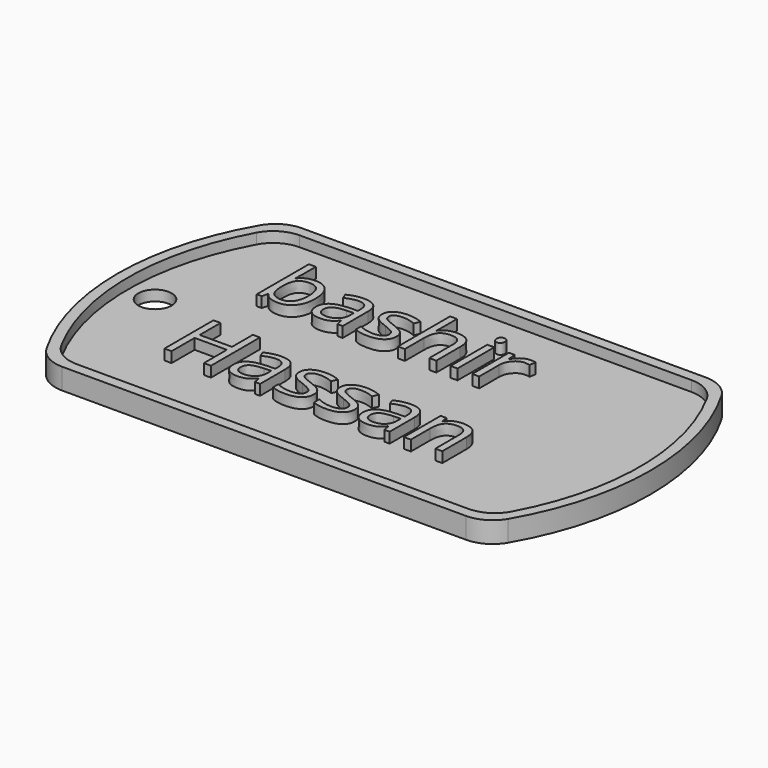
from build123d import *

# Parameters (mm, degrees)
F1_DEPTH     = 1
F3_DEPTH     = 1
F4_R         = 1.5875
F5_DEPTH     = 1
F6_TEXT_SIZE = 8.173513278
F7_DEPTH     = 1


# Not quite as in the source:
# - Text() gives the source's letters only with a copy of the font that has no kerning and outlines rounded to 1/6400 em; it was checked with that copy


with BuildPart() as f1:
    # F0 (on Top) → F1 (new body)
    with BuildSketch(Plane.XY):
        with BuildLine():
            ThreePointArc((-19.2474145991, 14.2875), (-20.8349145991, 13.862130657), (-21.9970452561, 12.7))
            ThreePointArc((-21.9970452561, 12.7), (-25.4, 0), (-21.9970452561, -12.7))
            ThreePointArc((-21.9970452561, -12.7), (-20.8349145991, -13.862130657), (-19.2474145991, -14.2875))
            Line((-19.2474145991, -14.2875), (19.2474145991, -14.2875))
            ThreePointArc((19.2474145991, -14.2875), (20.8349145991, -13.862130657), (21.9970452561, -12.7))
            ThreePointArc((21.9970452561, -12.7), (25.4, 0), (21.9970452561, 12.7))
            ThreePointArc((21.9970452561, 12.7), (20.8349145991, 13.862130657), (19.2474145991, 14.2875))
            Line((19.2474145991, 14.2875), (-19.2474145991, 14.2875))
        make_face()
    extrude(amount=F1_DEPTH)

    # F2 (on face) → F3 (join)
    with BuildSketch(Plane.XY.offset(1)):
        with BuildLine():
            Line((19.2474145991, 14.2875), (-19.2474145991, 14.2875))
            ThreePointArc((-19.2474145991, 14.2875), (-20.8349145991, 13.862130657), (-21.9970452561, 12.7))
            ThreePointArc((-21.9970452561, 12.7), (-25.4, 0), (-21.9970452561, -12.7))
            ThreePointArc((-21.9970452561, -12.7), (-20.8349145991, -13.862130657), (-19.2474145991, -14.2875))
            Line((-19.2474145991, -14.2875), (19.2474145991, -14.2875))
            ThreePointArc((19.2474145991, -14.2875), (20.8349145991, -13.862130657), (21.9970452561, -12.7))
            ThreePointArc((21.9970452561, -12.7), (25.4, 0), (21.9970452561, 12.7))
            ThreePointArc((21.9970452561, 12.7), (20.8349145991, 13.862130657), (19.2474145991, 14.2875))
        make_face()
        with BuildLine():
            ThreePointArc((-21.4526124879, 11.6252061249), (-20.2856017842, 12.8404540819), (-18.6611352482, 13.2875))
            Line((-18.6611352482, 13.2875), (18.6611352482, 13.2875))
            ThreePointArc((18.6611352482, 13.2875), (20.2856017842, 12.8404540819), (21.4526124879, 11.6252061249))
            ThreePointArc((21.4526124879, 11.6252061249), (24.4, 0), (21.4526124879, -11.6252061249))
            ThreePointArc((21.4526124879, -11.6252061249), (20.2856017842, -12.8404540819), (18.6611352482, -13.2875))
            Line((18.6611352482, -13.2875), (-18.6611352482, -13.2875))
            ThreePointArc((-18.6611352482, -13.2875), (-20.2856017842, -12.8404540819), (-21.4526124879, -11.6252061249))
            ThreePointArc((-21.4526124879, -11.6252061249), (-24.4, 0), (-21.4526124879, 11.6252061249))
        make_face(mode=Mode.SUBTRACT)
    extrude(amount=F3_DEPTH)

    # F4 (on face) → F5 (cut)
    with BuildSketch(Plane.XY.offset(1)):
        with Locations((-21.821282804, 0)):
            Circle(F4_R)
    extrude(amount=-F5_DEPTH, mode=Mode.SUBTRACT)

    # F6 (on face) → F7 (join)
    with BuildSketch(Plane.XY.offset(1)):
        with Locations((-15.9255936742, 3.8701156154)):
            Text('bashir', F6_TEXT_SIZE, font='Open Sans', text_align=(TextAlign.LEFT, TextAlign.BOTTOM))
        with Locations((-15.9255936742, -7.2458624426)):
            Text('Hassan', F6_TEXT_SIZE, font='Open Sans', text_align=(TextAlign.LEFT, TextAlign.BOTTOM))
    extrude(amount=F7_DEPTH)


solid = f1.part
